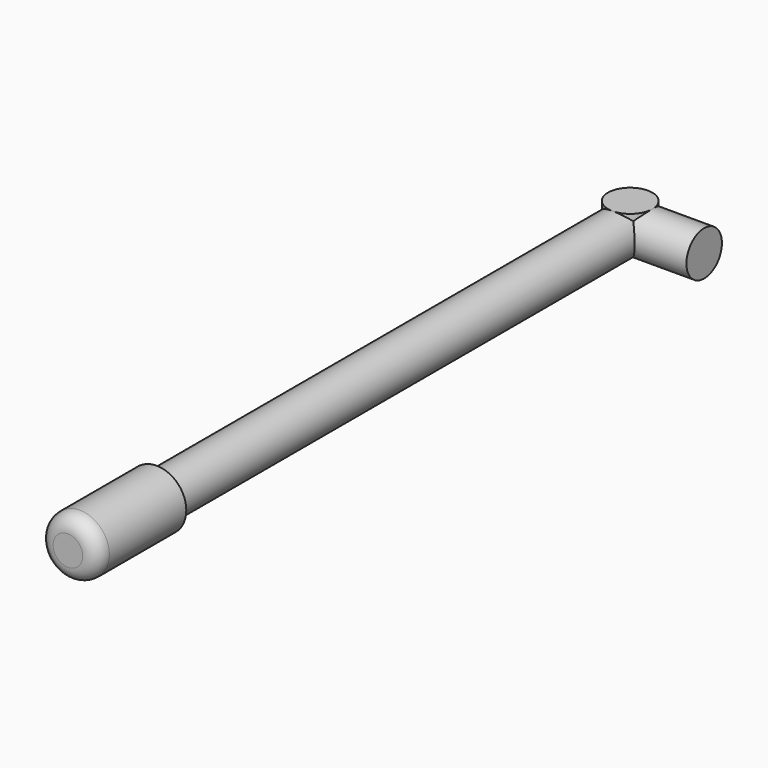
from build123d import *

# Parameters (mm, degrees)
F0_R     = 3
F1_DEPTH = 80
F2_R     = 4
F2_R_2   = 3
F3_DEPTH = 15
F4_R     = 2
F5_R     = 3
F6_DEPTH = 10
F7_R     = 3
F8_DEPTH = 3
F9_DEPTH = 3
F10_R    = 2.9999


# Not quite as in the source:
# - a fillet or chamfer is up to 0.001 mm smaller than in the source, because OpenCascade refuses the exact size


with BuildPart() as f1:
    # F0 (on Front) → F1 (new body)
    with BuildSketch(Plane.XZ):
        Circle(F0_R)
    extrude(amount=F1_DEPTH)

    # F2 (on face) → F3 (join)
    with BuildSketch(Plane.XZ.offset(80)):
        Circle(F2_R)
        Circle(F2_R_2, mode=Mode.SUBTRACT)
        Circle(F2_R_2)
    extrude(amount=F3_DEPTH)

    # F4
    f4_edges = [f1.edges().sort_by_distance(p)[0] for p in [
        (-4, -95, 0),
    ]]
    fillet(f4_edges, radius=F4_R)

    # F5 (on Right) → F6 (join)
    with BuildSketch(Plane.YZ):
        Circle(F5_R)
    extrude(amount=F6_DEPTH)

    # F7 (on Top) → F8 (join)
    with BuildSketch(Plane.XY):
        Circle(F7_R)
    extrude(amount=F8_DEPTH)

    # F9 (add): a face of the model
    f9_faces = [f1.faces().sort_by_distance(p)[0] for p in [
        (-1.2732395447, 1.2732395447, 0),
    ]]
    extrude(f9_faces, amount=F9_DEPTH)

    # F10 (radius 3 in the source; OpenCascade refuses exactly that, so slightly less here)
    f10_edges = [f1.edges().sort_by_distance(p)[0] for p in [
        (-2.12132, 2.12132, -3),
    ]]
    fillet(f10_edges, radius=F10_R)


solid = f1.part
